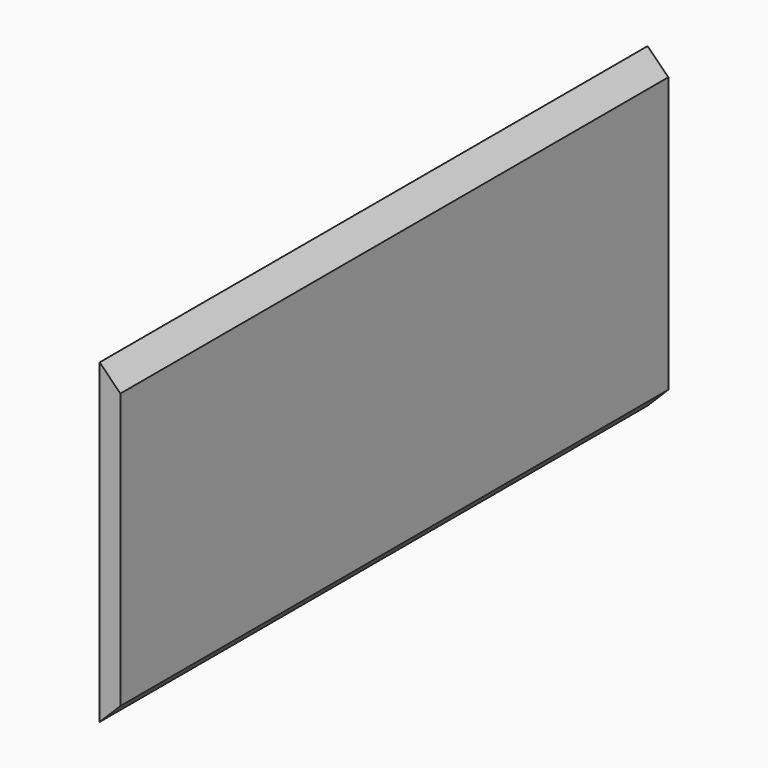
from build123d import *

# Parameters (mm, degrees)
F0_W     = 595
F0_H     = 275
F1_DEPTH = 18
F2_SIZE  = 17.99999


# Not quite as in the source:
# - a fillet or chamfer is up to 0.001 mm smaller than in the source, because OpenCascade refuses the exact size


with BuildPart() as f1:
    # F0 (on Right) → F1 (new body)
    with BuildSketch(Plane.YZ):
        Rectangle(F0_W, F0_H)
    extrude(amount=F1_DEPTH)

    # F2 (size 18 in the source; OpenCascade refuses exactly that, so slightly less here)
    f2_edges = [f1.edges().sort_by_distance(p)[0] for p in [
        (18, 0, 137.5),
        (18, 0, -137.5),
    ]]
    chamfer(f2_edges, length=F2_SIZE)


solid = f1.part
